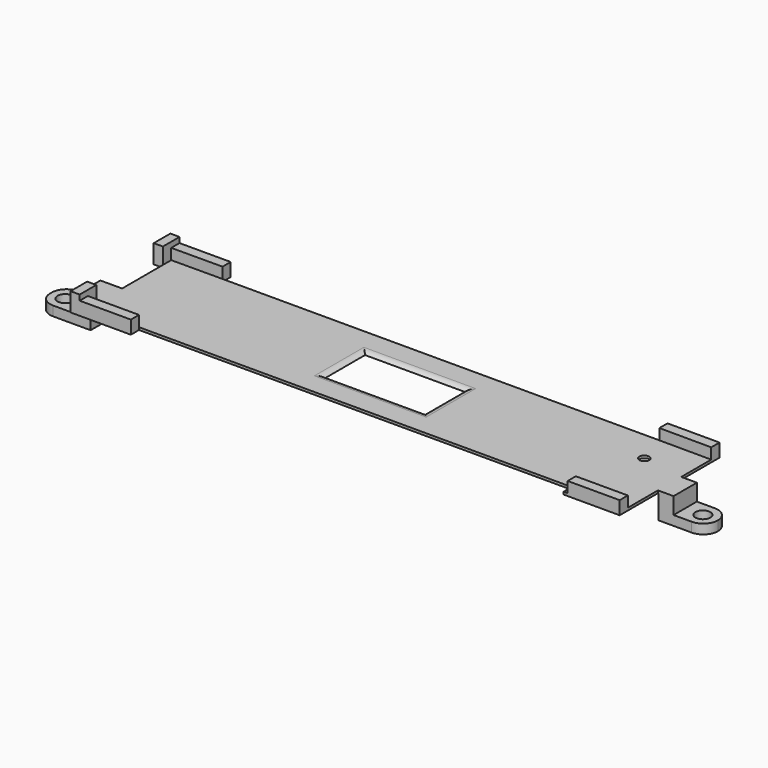
from build123d import *

# Parameters (mm, degrees)
F0_W          = 24
F0_H          = 12
F1_DEPTH      = 4.5
F2_W          = 134.0499658869
F2_H          = 37.3212727123
F3_DEPTH      = 1.3
F5_DEPTH      = 2.6
F6_R          = 1.8
F6_R_2        = 1.8546222436
F7_DEPTH      = 6.3
F8_W          = 131.4748737342
F8_H          = 57.6514146297
F9_DEPTH      = 5.7
F10_R         = 1.175
F11_DEPTH     = 2
F12_R         = 1.8546222436
F12_R_2       = 1.8
F13_DEPTH     = 4
F14_T1_DEPTH  = 24
F14_T3_DEPTH  = 12
F14_T9_DEPTH  = 15.5707142143
F14_T13_DEPTH = 27.5707142143
F14_T20_DEPTH = 27.5707142143
F14_T24_DEPTH = 15.5707142143
F14_T31_DEPTH = 15.5707142143
F14_T35_DEPTH = 27.5707142143
F14_T42_DEPTH = 27.5707142143
F14_T46_DEPTH = 15.5707142143


# Not quite as in the source:
# - a fillet or chamfer that OpenCascade refuses, or shapes differently, is made with other operations: its cross-section is extruded or revolved along the edge and cut away or added


with BuildPart() as f1:
    # F0 (on Top) → F1 (new body)
    with BuildSketch(Plane.XY):
        Polygon((-51.5, 15), (-66, 15), (-66, 10), (-63.8, 10), (-63.8, -10), (-66, -10), (-66, -15), (-51.5, -15), (-51.5, -12.55), (52.5, -12.55), (52.5, -15), (66, -15), (66, 15), (53.5, 15), (53.5, 12.55), (-51.5, 12.55), align=None)
        Rectangle(F0_W, F0_H, mode=Mode.SUBTRACT)
    extrude(amount=F1_DEPTH)

    # F2 (on face) → F3 (cut)
    with BuildSketch(Plane.XY.offset(4.5)):
        with Locations((3.2249829435, -1.1242744513)):
            Rectangle(F2_W, F2_H)
    extrude(amount=-F3_DEPTH, mode=Mode.SUBTRACT)

    # F4 (on face) → F5 (cut)
    with BuildSketch(Plane.XY.offset(3.2)):
        Polygon((-63.8, 12.5), (-63.8, -12.55), (-51.5, -12.55), (-51.5, -30.0471726805), (53.5, -30.0471726805), (53.5, -12.55), (68.7586962298, -12.55), (68.7586962298, 12.5), (53.5, 12.55), (53.5, 21.0785120726), (-51.5, 21.0785120726), (-51.5, 12.55), align=None)
    extrude(amount=-F5_DEPTH, mode=Mode.SUBTRACT)

    # F6 (on face) → F7 (join)
    with BuildSketch(Plane.XY.offset(0.6)):
        with BuildLine():
            Line((66, 3.5), (66, -3.5))
            Line((66, -3.5), (74.1, -3.5))
            ThreePointArc((74.1, -3.5), (76.5748737342, -2.4748737342), (77.6, 0))
            ThreePointArc((77.6, 0), (76.5748737342, 2.4748737342), (74.1, 3.5))
            Line((74.1, 3.5), (66, 3.5))
        make_face()
        with Locations((74, 0)):
            Circle(F6_R, mode=Mode.SUBTRACT)
        with BuildLine():
            Line((-74.4, -9.75), (-63.8, -9.75))
            Line((-63.8, -9.75), (-63.8, -2.25))
            Line((-63.8, -2.25), (-74.4, -2.25))
            ThreePointArc((-74.4, -2.25), (-76.8748737342, -3.2751262658), (-77.9, -5.75))
            Line((-77.9, -5.75), (-77.9, -6.25))
            ThreePointArc((-77.9, -6.25), (-76.8748737342, -8.7248737342), (-74.4, -9.75))
        make_face()
        with Locations((-74.35, -6.136629995)):
            Circle(F6_R_2, mode=Mode.SUBTRACT)
    extrude(amount=-F7_DEPTH)

    # F8 (on face) → F9 (cut, through all)
    with BuildSketch(Plane(origin=(0, 0, -5.7), x_dir=(1, 0, 0), z_dir=(0, 0, -1))):
        with Locations((0.3625631329, -2.5597326458)):
            Rectangle(F8_W, F8_H)
    extrude(amount=-F9_DEPTH, mode=Mode.SUBTRACT)

    # F10 (on face) → F11 (cut)
    with BuildSketch(Plane(origin=(0, 0, 0), x_dir=(1, 0, 0), z_dir=(0, 0, -1))):
        with Locations((55.875, -5.075)):
            Circle(F10_R)
    extrude(amount=-F11_DEPTH, mode=Mode.SUBTRACT)

    # F12 (on face) → F13 (cut)
    with BuildSketch(Plane.XY.offset(0.6)):
        with BuildLine():
            Line((-69.0248737342, -9.75), (-69.0248737342, -2.25))
            Line((-69.0248737342, -2.25), (-74.4, -2.25))
            ThreePointArc((-74.4, -2.25), (-76.8748737342, -3.2751262658), (-77.9, -5.75))
            Line((-77.9, -5.75), (-77.9, -6.25))
            ThreePointArc((-77.9, -6.25), (-76.8748737342, -8.7248737342), (-74.4, -9.75))
            Line((-74.4, -9.75), (-69.0248737342, -9.75))
        make_face()
        with Locations((-74.35, -6.136629995)):
            Circle(F12_R, mode=Mode.SUBTRACT)
        with BuildLine():
            Line((74.1, 3.5), (69.75, 3.5))
            Line((69.75, 3.5), (69.75, -3.5))
            Line((69.75, -3.5), (74.1, -3.5))
            ThreePointArc((74.1, -3.5), (77.6, 0), (74.1, 3.5))
        make_face()
        with Locations((74, 0)):
            Circle(F12_R_2, mode=Mode.SUBTRACT)
    extrude(amount=-F13_DEPTH, mode=Mode.SUBTRACT)

    # F14: fillet of radius 2 on 4 edges, made by hand

    # F14_s2 → F14_t1 (cut)
    with BuildSketch(Plane.YZ.offset(-12)):
        with BuildLine():
            ThreePointArc((6, 0), (6.6536890165, 0.4439088915), (7.4282856857, 0.6))
            Line((7.4282856857, 0.6), (6, 0.6))
            Line((6, 0.6), (6, 0))
        make_face()
        with BuildLine():
            ThreePointArc((-6, 0), (-6.6536890165, 0.4439088915), (-7.4282856857, 0.6))
            Line((-7.4282856857, 0.6), (-6, 0.6))
            Line((-6, 0.6), (-6, 0))
        make_face()
    extrude(amount=F14_T1_DEPTH, mode=Mode.SUBTRACT)

    # F14_s4 → F14_t3 (cut)
    with BuildSketch(Plane.XZ.offset(-6)):
        with BuildLine():
            ThreePointArc((-12, 0), (-12.6536890165, 0.4439088915), (-13.4282856857, 0.6))
            Line((-13.4282856857, 0.6), (-12, 0.6))
            Line((-12, 0.6), (-12, 0))
        make_face()
        with BuildLine():
            ThreePointArc((12, 0), (12.6536890165, 0.4439088915), (13.4282856857, 0.6))
            Line((13.4282856857, 0.6), (12, 0.6))
            Line((12, 0.6), (12, 0))
        make_face()
    extrude(amount=F14_T3_DEPTH, mode=Mode.SUBTRACT)


with BuildPart() as f14_tool7:
    # F14_s8 → F14_t9 (new body)
    with BuildSketch(Plane.XZ.offset(6)):
        with BuildLine():
            ThreePointArc((-12, 0), (-12.6536890165, 0.4439088915), (-13.4282856857, 0.6))
            Line((-13.4282856857, 0.6), (-12, 0.6))
            Line((-12, 0.6), (-12, 0))
        make_face()
    extrude(amount=-F14_T9_DEPTH)

    split(bisect_by=Plane.XZ.offset(-6), keep=Keep.BOTTOM)


with BuildPart() as f14_tool11:
    # F14_s12 → F14_t13 (new body)
    with BuildSketch(Plane.YZ.offset(-15.5707142143)):
        with BuildLine():
            ThreePointArc((6, 0), (6.6536890165, 0.4439088915), (7.4282856857, 0.6))
            Line((7.4282856857, 0.6), (6, 0.6))
            Line((6, 0.6), (6, 0))
        make_face()
    extrude(amount=F14_T13_DEPTH)

    split(bisect_by=Plane.YZ.offset(-12), keep=Keep.BOTTOM)


with BuildPart() as f14_tool7_1:
    add(f14_tool7.part)

    # F14_t15: intersect F14_tool11
    add(f14_tool11.part, mode=Mode.INTERSECT)


with BuildPart() as f1_1:
    add(f1.part)

    # F14_t5: cut F14_tool7
    add(f14_tool7_1.part, mode=Mode.SUBTRACT)


with BuildPart() as f14_tool18:
    # F14_s19 → F14_t20 (new body)
    with BuildSketch(Plane.YZ.offset(-12)):
        with BuildLine():
            ThreePointArc((6, 0), (6.6536890165, 0.4439088915), (7.4282856857, 0.6))
            Line((7.4282856857, 0.6), (6, 0.6))
            Line((6, 0.6), (6, 0))
        make_face()
    extrude(amount=F14_T20_DEPTH)

    split(bisect_by=Plane.YZ.offset(12), keep=Keep.TOP)


with BuildPart() as f14_tool22:
    # F14_s23 → F14_t24 (new body)
    with BuildSketch(Plane.XZ.offset(-9.5707142143)):
        with BuildLine():
            ThreePointArc((12, 0), (12.6536890165, 0.4439088915), (13.4282856857, 0.6))
            Line((13.4282856857, 0.6), (12, 0.6))
            Line((12, 0.6), (12, 0))
        make_face()
    extrude(amount=F14_T24_DEPTH)

    split(bisect_by=Plane.XZ.offset(-6), keep=Keep.BOTTOM)


with BuildPart() as f14_tool18_1:
    add(f14_tool18.part)

    # F14_t26: intersect F14_tool22
    add(f14_tool22.part, mode=Mode.INTERSECT)


with BuildPart() as f1_2:
    add(f1_1.part)

    # F14_t16: cut F14_tool18
    add(f14_tool18_1.part, mode=Mode.SUBTRACT)


with BuildPart() as f14_tool29:
    # F14_s30 → F14_t31 (new body)
    with BuildSketch(Plane.XZ.offset(9.5707142143)):
        with BuildLine():
            ThreePointArc((-12, 0), (-12.6536890165, 0.4439088915), (-13.4282856857, 0.6))
            Line((-13.4282856857, 0.6), (-12, 0.6))
            Line((-12, 0.6), (-12, 0))
        make_face()
    extrude(amount=-F14_T31_DEPTH)

    split(bisect_by=Plane.XZ.offset(6), keep=Keep.TOP)


with BuildPart() as f14_tool33:
    # F14_s34 → F14_t35 (new body)
    with BuildSketch(Plane.YZ.offset(12)):
        with BuildLine():
            ThreePointArc((-6, 0), (-6.6536890165, 0.4439088915), (-7.4282856857, 0.6))
            Line((-7.4282856857, 0.6), (-6, 0.6))
            Line((-6, 0.6), (-6, 0))
        make_face()
    extrude(amount=-F14_T35_DEPTH)

    split(bisect_by=Plane.YZ.offset(-12), keep=Keep.BOTTOM)


with BuildPart() as f14_tool29_1:
    add(f14_tool29.part)

    # F14_t37: intersect F14_tool33
    add(f14_tool33.part, mode=Mode.INTERSECT)


with BuildPart() as f1_3:
    add(f1_2.part)

    # F14_t27: cut F14_tool29
    add(f14_tool29_1.part, mode=Mode.SUBTRACT)


with BuildPart() as f14_tool40:
    # F14_s41 → F14_t42 (new body)
    with BuildSketch(Plane.YZ.offset(15.5707142143)):
        with BuildLine():
            ThreePointArc((-6, 0), (-6.6536890165, 0.4439088915), (-7.4282856857, 0.6))
            Line((-7.4282856857, 0.6), (-6, 0.6))
            Line((-6, 0.6), (-6, 0))
        make_face()
    extrude(amount=-F14_T42_DEPTH)

    split(bisect_by=Plane.YZ.offset(12), keep=Keep.TOP)


with BuildPart() as f14_tool44:
    # F14_s45 → F14_t46 (new body)
    with BuildSketch(Plane.XZ.offset(-6)):
        with BuildLine():
            ThreePointArc((12, 0), (12.6536890165, 0.4439088915), (13.4282856857, 0.6))
            Line((13.4282856857, 0.6), (12, 0.6))
            Line((12, 0.6), (12, 0))
        make_face()
    extrude(amount=F14_T46_DEPTH)

    split(bisect_by=Plane.XZ.offset(6), keep=Keep.TOP)


with BuildPart() as f14_tool40_1:
    add(f14_tool40.part)

    # F14_t48: intersect F14_tool44
    add(f14_tool44.part, mode=Mode.INTERSECT)


with BuildPart() as f1_4:
    add(f1_3.part)

    # F14_t38: cut F14_tool40
    add(f14_tool40_1.part, mode=Mode.SUBTRACT)


solid = f1_4.part
